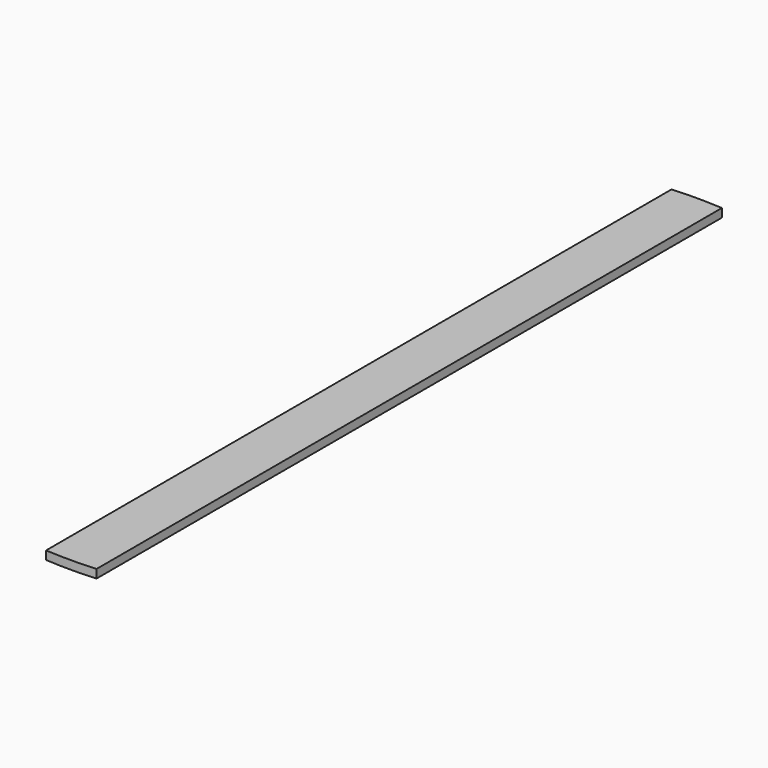
from build123d import *

# Parameters (mm, degrees)
F1_DEPTH = 38


# Not quite as in the source:
# - a feature names something its author has since deleted; it is built from what else it names


with BuildPart() as f1:
    # F0 (on Top) → F1 (new body)
    with BuildSketch(Plane.XY):
        with BuildLine():
            ThreePointArc((113.4371591732, 3396.0578373807), (0.9391016735, 3399.738023894), (-111.5628408268, 3396.1785790418))
            Line((-111.5628408268, 3396.1785790418), (-111.5628408268, -96.702027304))
            ThreePointArc((-111.5628408268, -96.702027304), (0.9391016735, -100.2614721563), (113.4371591732, -96.5812856429))
            Line((113.4371591732, -96.5812856429), (113.4371591732, 3396.0578373807))
        make_face()
    extrude(amount=F1_DEPTH)


solid = f1.part
